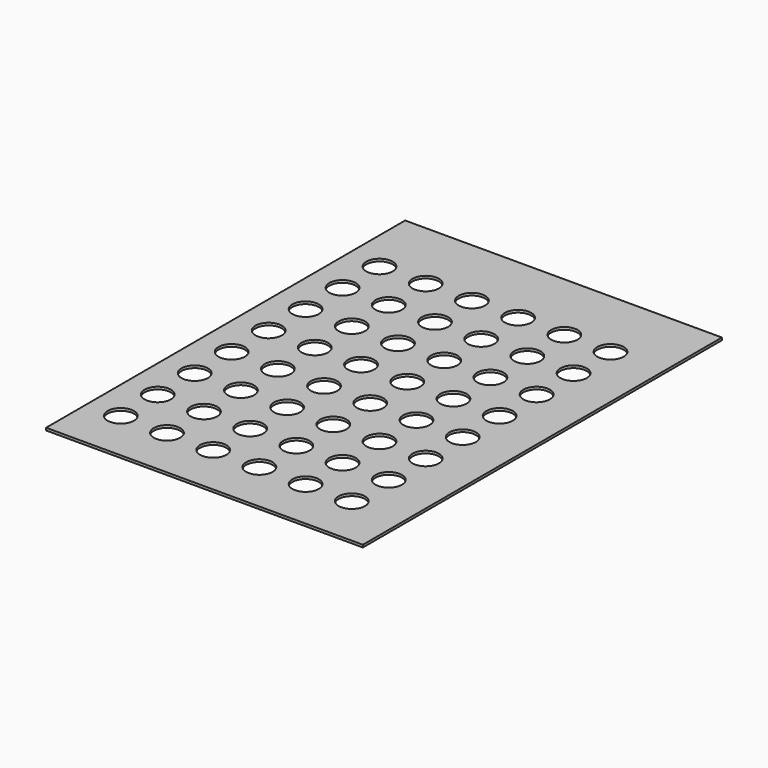
from build123d import *

# Parameters (mm, degrees)
F0_W     = 609.6
F0_H     = 863.6
F0_R     = 25.4
F1_DEPTH = 4.7625


# Not quite as in the source:
# - a length typed as a fraction of an inch, garbled in the dataset ("3 / 203.2 mm" for 3/8 in), is restored


with BuildPart() as f1:
    # F0 (on Top) → F1 (new body)
    with BuildSketch(Plane.XY):
        with Locations((-241.5563351989, 354.9824055314)):
            Rectangle(F0_W, F0_H)
        with Locations((-482.8563351989, 23.5082199097)):
            Circle(F0_R, mode=Mode.SUBTRACT)
        with Locations((-393.9563351989, 23.5082199097)):
            Circle(F0_R, mode=Mode.SUBTRACT)
        with Locations((-482.8563351989, 112.4082199097)):
            Circle(F0_R, mode=Mode.SUBTRACT)
        with Locations((-393.9563351989, 112.4082199097)):
            Circle(F0_R, mode=Mode.SUBTRACT)
        with Locations((-305.0563351989, 23.5082199097)):
            Circle(F0_R, mode=Mode.SUBTRACT)
        with Locations((-305.0563351989, 112.4082199097)):
            Circle(F0_R, mode=Mode.SUBTRACT)
        with Locations((-482.8563351989, 201.3082199097)):
            Circle(F0_R, mode=Mode.SUBTRACT)
        with Locations((-393.9563351989, 201.3082199097)):
            Circle(F0_R, mode=Mode.SUBTRACT)
        with Locations((-482.8563351989, 290.2082199097)):
            Circle(F0_R, mode=Mode.SUBTRACT)
        with Locations((-393.9563351989, 290.2082199097)):
            Circle(F0_R, mode=Mode.SUBTRACT)
        with Locations((-305.0563351989, 201.3082199097)):
            Circle(F0_R, mode=Mode.SUBTRACT)
        with Locations((-305.0563351989, 290.2082199097)):
            Circle(F0_R, mode=Mode.SUBTRACT)
        with Locations((-216.1563351989, 23.5082199097)):
            Circle(F0_R, mode=Mode.SUBTRACT)
        with Locations((-127.2563351989, 23.5082199097)):
            Circle(F0_R, mode=Mode.SUBTRACT)
        with Locations((-216.1563351989, 112.4082199097)):
            Circle(F0_R, mode=Mode.SUBTRACT)
        with Locations((-127.2563351989, 112.4082199097)):
            Circle(F0_R, mode=Mode.SUBTRACT)
        with Locations((-38.3563351989, 23.5082199097)):
            Circle(F0_R, mode=Mode.SUBTRACT)
        with Locations((-38.3563351989, 112.4082199097)):
            Circle(F0_R, mode=Mode.SUBTRACT)
        with Locations((-216.1563351989, 201.3082199097)):
            Circle(F0_R, mode=Mode.SUBTRACT)
        with Locations((-127.2563351989, 201.3082199097)):
            Circle(F0_R, mode=Mode.SUBTRACT)
        with Locations((-216.1563351989, 290.2082199097)):
            Circle(F0_R, mode=Mode.SUBTRACT)
        with Locations((-127.2563351989, 290.2082199097)):
            Circle(F0_R, mode=Mode.SUBTRACT)
        with Locations((-38.3563351989, 201.3082199097)):
            Circle(F0_R, mode=Mode.SUBTRACT)
        with Locations((-38.3563351989, 290.2082199097)):
            Circle(F0_R, mode=Mode.SUBTRACT)
        with Locations((-482.8563351989, 379.1082199097)):
            Circle(F0_R, mode=Mode.SUBTRACT)
        with Locations((-393.9563351989, 379.1082199097)):
            Circle(F0_R, mode=Mode.SUBTRACT)
        with Locations((-482.8563351989, 468.0082199097)):
            Circle(F0_R, mode=Mode.SUBTRACT)
        with Locations((-482.8563351989, 556.9082199097)):
            Circle(F0_R, mode=Mode.SUBTRACT)
        with Locations((-393.9563351989, 468.0082199097)):
            Circle(F0_R, mode=Mode.SUBTRACT)
        with Locations((-393.9563351989, 556.9082199097)):
            Circle(F0_R, mode=Mode.SUBTRACT)
        with Locations((-305.0563351989, 379.1082199097)):
            Circle(F0_R, mode=Mode.SUBTRACT)
        with Locations((-305.0563351989, 468.0082199097)):
            Circle(F0_R, mode=Mode.SUBTRACT)
        with Locations((-305.0563351989, 556.9082199097)):
            Circle(F0_R, mode=Mode.SUBTRACT)
        with Locations((-482.8563351989, 645.8082199097)):
            Circle(F0_R, mode=Mode.SUBTRACT)
        with Locations((-393.9563351989, 645.8082199097)):
            Circle(F0_R, mode=Mode.SUBTRACT)
        with Locations((-305.0563351989, 645.8082199097)):
            Circle(F0_R, mode=Mode.SUBTRACT)
        with Locations((-216.1563351989, 379.1082199097)):
            Circle(F0_R, mode=Mode.SUBTRACT)
        with Locations((-127.2563351989, 379.1082199097)):
            Circle(F0_R, mode=Mode.SUBTRACT)
        with Locations((-216.1563351989, 468.0082199097)):
            Circle(F0_R, mode=Mode.SUBTRACT)
        with Locations((-216.1563351989, 556.9082199097)):
            Circle(F0_R, mode=Mode.SUBTRACT)
        with Locations((-127.2563351989, 468.0082199097)):
            Circle(F0_R, mode=Mode.SUBTRACT)
        with Locations((-127.2563351989, 556.9082199097)):
            Circle(F0_R, mode=Mode.SUBTRACT)
        with Locations((-38.3563351989, 379.1082199097)):
            Circle(F0_R, mode=Mode.SUBTRACT)
        with Locations((-38.3563351989, 468.0082199097)):
            Circle(F0_R, mode=Mode.SUBTRACT)
        with Locations((-38.3563351989, 556.9082199097)):
            Circle(F0_R, mode=Mode.SUBTRACT)
        with Locations((-216.1563351989, 645.8082199097)):
            Circle(F0_R, mode=Mode.SUBTRACT)
        with Locations((-127.2563351989, 645.8082199097)):
            Circle(F0_R, mode=Mode.SUBTRACT)
        with Locations((-38.3563351989, 645.8082199097)):
            Circle(F0_R, mode=Mode.SUBTRACT)
    extrude(amount=F1_DEPTH)


solid = f1.part
